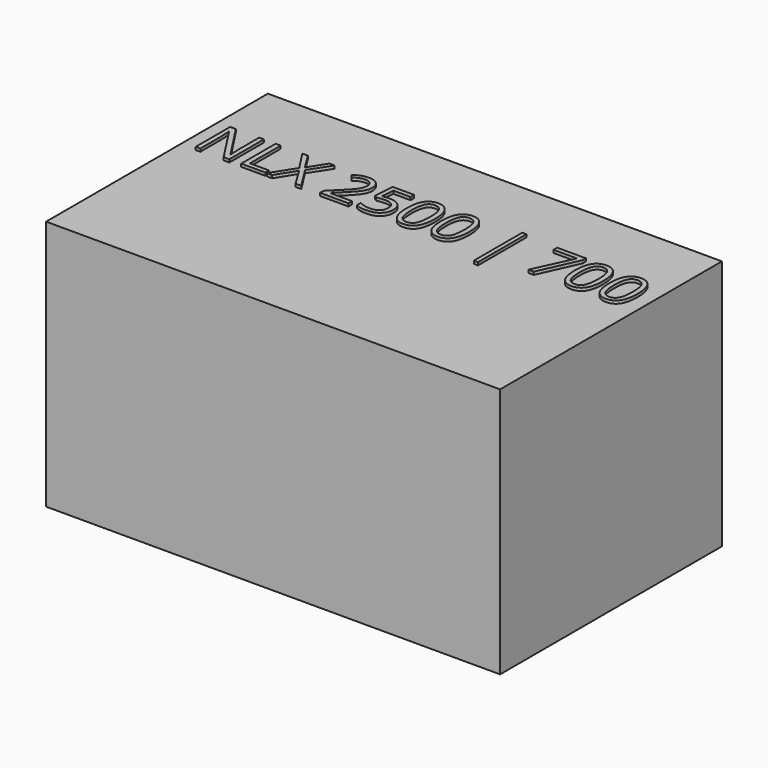
from build123d import *

# Parameters (mm, degrees)
F0_W         = 3980.18
F0_H         = 2430.78
F1_DEPTH     = 2199.64
F2_TEXT_SIZE = 529.3389775317
F3_DEPTH     = 25.4


# Not quite as in the source:
# - Text() gives the source's letters only with a copy of the font that has no kerning and outlines rounded to 1/6400 em; it was checked with that copy


with BuildPart() as f1:
    # F0 (on Top) → F1 (new body)
    with BuildSketch(Plane.XY):
        Rectangle(F0_W, F0_H)
    extrude(amount=F1_DEPTH)

    # F2 (on face) → F3 (join)
    with BuildSketch(Plane.XY.offset(2199.64)):
        with Locations((-1905, 252.9277955724)):
            Text('NLX 2500 | 700', F2_TEXT_SIZE, font='Open Sans', text_align=(TextAlign.LEFT, TextAlign.BOTTOM))
    extrude(amount=F3_DEPTH)


solid = f1.part
